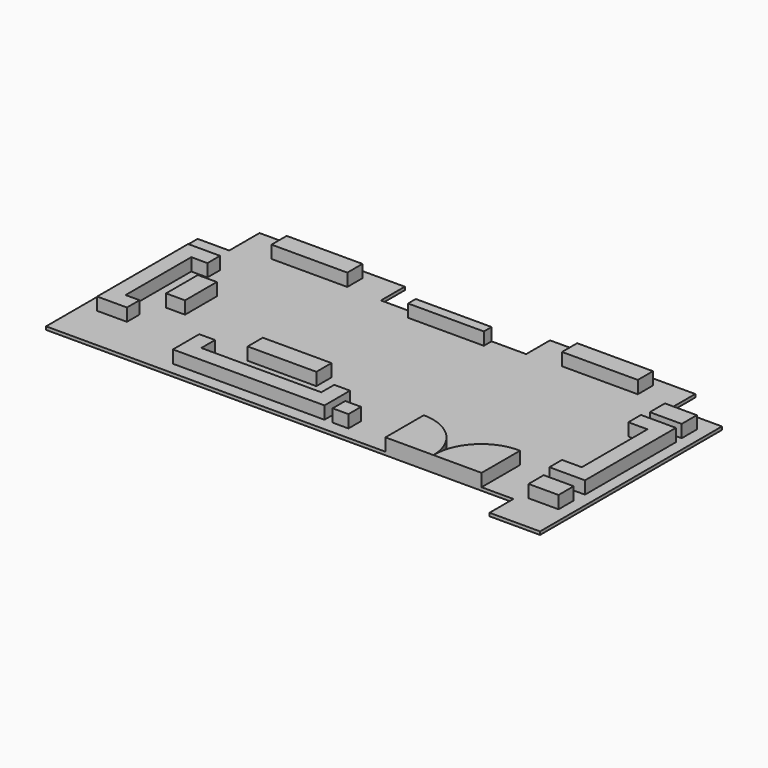
from build123d import *

# Parameters (mm, degrees)
F1_DEPTH = 50
F2_W     = 1200
F2_H     = 300
F2_W_2   = 300
F2_H_2   = 629.1752159595
F2_W_3   = 1087.7267122269
F2_W_4   = 250
F2_H_3   = 250
F2_H_4   = 152.9987954981
F2_W_5   = 504.9269199371
F2_W_6   = 474.6313095093
F3_DEPTH = 200
F4_DEPTH = 200


# Not quite as in the source:
# - a feature names something its author has since deleted; it is built from what else it names


with BuildPart() as f1:
    # F0 (on Top) → F1 (new body)
    with BuildSketch(Plane.XY):
        Polygon((-4707.8431632393, 1513.8580155657), (-4707.8431632393, -1486.1419844343), (2692.1568367607, -1486.1419844343), (2692.1568367607, -1958.4740257375), (3492.1568367607, -1958.4740257375), (3492.1568367607, 1641.5259742625), (2692.1568367607, 1641.5259742625), (2692.1568367607, 2113.8580155657), (392.1568367607, 2113.8580155657), (392.1568367607, 1641.5259742625), (-1907.8431632393, 1641.5259742625), (-1907.8431632393, 2113.8580155657), (-4207.8431632393, 2113.8580155657), (-4207.8431632393, 1513.8580155657), align=None)
    extrude(amount=F1_DEPTH)

    # F2 (on face) → F3 (join)
    with BuildSketch(Plane.XY.offset(50)):
        with Locations((-3057.8431632393, 1813.8580155657)):
            Rectangle(F2_W, F2_H)
        Polygon((-3967.6023748444, 782.182643881), (-3967.6023748444, 1032.182643881), (-4473.3698458788, 1032.182643881), (-4473.3698458788, -767.817356119), (-4002.1681580892, -767.817356119), (-4002.1681580892, -517.817356119), (-4223.3698458788, -517.817356119), (-4223.3698458788, 782.182643881), align=None)
        with Locations((-3710.9555244446, 144.9798196554)):
            Rectangle(F2_W_2, F2_H_2)
        Polygon((-2607.132434845, -766.7910456657), (-2857.132434845, -767.817356119), (-2857.132434845, -1289.3264293671), (-457.132434845, -1289.3264293671), (-457.132434845, -783.3907008171), (-707.132434845, -783.3907008171), (-707.132434845, -1039.3264293671), (-2607.132434845, -1039.3264293671), align=None)
        with Locations((-1641.4379477501, -499.4871973991)):
            Rectangle(F2_W_3, F2_H)
        with Locations((-204.7675848007, -1161.3585650921)):
            Rectangle(F2_W_4, F2_H_3)
        with Locations((-755.6409478188, 1565.0265765134)):
            Rectangle(F2_W, F2_H_4)
        with Locations((3048.9259958267, 1233.1605195999)):
            Rectangle(F2_W_5, F2_H)
        Polygon((3311.5372657776, 956.2834382057), (2758.581161499, 956.2834382057), (2758.581161499, 706.2834382057), (3061.5372657776, 706.2834382057), (3061.5372657776, -593.7165617943), (2748.4827041626, -593.7165617943), (2748.4827041626, -843.7165617943), (3311.5372657776, -843.7165617943), align=None)
        with Locations((3064.0738010406, -1204.2857170105)):
            Rectangle(F2_W_6, F2_H)
    extrude(amount=F3_DEPTH)

    # F2 (on face) → F4 (join)
    with BuildSketch(Plane.XY.offset(50)):
        with Locations((-3057.8431632393, 1813.8580155657)):
            Rectangle(F2_W, F2_H)
        Polygon((-3967.6023748444, 782.182643881), (-3967.6023748444, 1032.182643881), (-4473.3698458788, 1032.182643881), (-4473.3698458788, -767.817356119), (-4002.1681580892, -767.817356119), (-4002.1681580892, -517.817356119), (-4223.3698458788, -517.817356119), (-4223.3698458788, 782.182643881), align=None)
        with Locations((-3710.9555244446, 144.9798196554)):
            Rectangle(F2_W_2, F2_H_2)
        Polygon((-2607.132434845, -766.7910456657), (-2857.132434845, -767.817356119), (-2857.132434845, -1289.3264293671), (-457.132434845, -1289.3264293671), (-457.132434845, -783.3907008171), (-707.132434845, -783.3907008171), (-707.132434845, -1039.3264293671), (-2607.132434845, -1039.3264293671), align=None)
        with Locations((-1641.4379477501, -499.4871973991)):
            Rectangle(F2_W_3, F2_H)
        with Locations((-204.7675848007, -1161.3585650921)):
            Rectangle(F2_W_4, F2_H_3)
        with Locations((-755.6409478188, 1565.0265765134)):
            Rectangle(F2_W, F2_H_4)
        with Locations((1542.1568367607, 1813.8580155657)):
            Rectangle(F2_W, F2_H)
        with Locations((3048.9259958267, 1233.1605195999)):
            Rectangle(F2_W_5, F2_H)
        Polygon((3311.5372657776, 956.2834382057), (2758.581161499, 956.2834382057), (2758.581161499, 706.2834382057), (3061.5372657776, 706.2834382057), (3061.5372657776, -593.7165617943), (2748.4827041626, -593.7165617943), (2748.4827041626, -843.7165617943), (3311.5372657776, -843.7165617943), align=None)
        with Locations((3064.0738010406, -1204.2857170105)):
            Rectangle(F2_W_6, F2_H)
        with BuildLine():
            Line((666.3535618782, -726.1419844343), (666.3535618782, -1486.1419844343))
            Line((666.3535618782, -1486.1419844343), (1426.3535618782, -1486.1419844343))
            ThreePointArc((1426.3535618782, -1486.1419844343), (1200.2233986174, -952.2721476951), (666.3535618782, -726.1419844343))
        make_face()
        with BuildLine():
            Line((1428.3535618782, -1486.1419844343), (2188.3535618782, -1486.1419844343))
            Line((2188.3535618782, -1486.1419844343), (2188.3535618782, -726.1419844343))
            ThreePointArc((2188.3535618782, -726.1419844343), (1642.4705952714, -940.2590178275), (1428.3535618782, -1486.1419844343))
        make_face()
    extrude(amount=F4_DEPTH)


solid = f1.part
